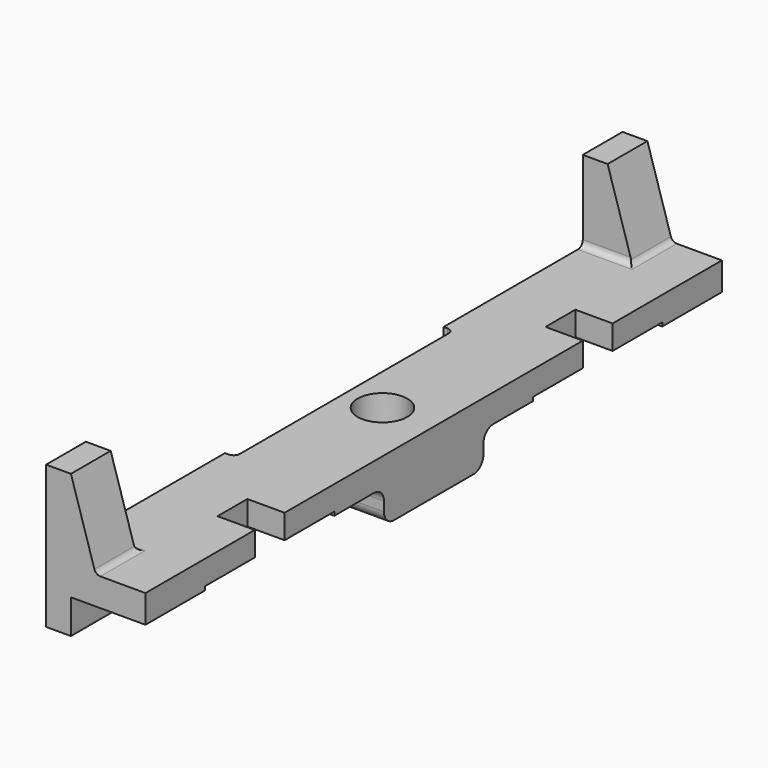
from build123d import *

# Parameters (mm, degrees)
F0_W      = 58
F0_H      = 5
F1_DEPTH  = 2
F2_W      = 13
F2_H      = 0.5
F3_DEPTH  = 0.8
F4_W      = 58
F4_H      = 2.25
F5_DEPTH  = 6
F6_W      = 6
F6_H      = 10
F7_DEPTH  = 2.75
F8_R      = 2
F9_DEPTH  = 4
F10_R     = 1
F12_DEPTH = 4
F13_W     = 22
F13_H     = 5
F14_DEPTH = 0.8
F15_R     = 0.5
F16_W     = 6.8
F16_H     = 13
F17_DEPTH = 0.3
F18_W     = 3
F18_H     = 3
F19_DEPTH = 1.95


# Not quite as in the source:
# - a pattern or mirror of a feature is missing from the dataset's text; its kind, count and spacing are read off the source's solid


with BuildPart() as f1:
    # F0 (on Right) → F1 (new body)
    with BuildSketch(Plane.YZ):
        Rectangle(F0_W, F0_H)
    extrude(amount=F1_DEPTH)

    # F2 (on face) → F3 (cut)
    with BuildSketch(Plane.YZ.offset(2)):
        with Locations((16.5, 0)):
            Rectangle(F2_W, F2_H)
        with Locations((-16.5, 0)):
            Rectangle(F2_W, F2_H)
    extrude(amount=-F3_DEPTH, mode=Mode.SUBTRACT)

    # F4 (on face) → F5 (join)
    with BuildSketch(Plane.YZ.offset(2)):
        with Locations((0, 1.375)):
            Rectangle(F4_W, F4_H)
    extrude(amount=F5_DEPTH)

    # F6 (on face) → F7 (join, through all)
    with BuildSketch(Plane(origin=(0, 0, 0.25), x_dir=(1, 0, 0), z_dir=(0, 0, -1))):
        with Locations((5, 0)):
            Rectangle(F6_W, F6_H)
    extrude(amount=F7_DEPTH)

    # F8 (on face) → F9 (cut)
    with BuildSketch(Plane.XY.offset(2.5)):
        with Locations((3.875, 0)):
            Circle(F8_R)
    extrude(amount=-F9_DEPTH, mode=Mode.SUBTRACT)

    # F10
    f10_edges = [f1.edges().sort_by_distance(p)[0] for p in [
        (5, -5, -2.5),
        (5, -5, 0.25),
        (5, 5, 0.25),
        (5, 5, -2.5),
    ]]
    fillet(f10_edges, radius=F10_R)

    # F11 (on face) → F12 (join)
    with BuildSketch(Plane(origin=(0, 29, 0), x_dir=(-1, 0, 0), z_dir=(0, 1, 0))):
        Polygon((-4, 2.5), (0, 2.5), (0, 9), (-2, 9), align=None)
    f12 = extrude(amount=-F12_DEPTH)

    # F12_copies: F12 across plane
    add(f12.mirror(Plane(origin=(0, 0, 0), x_dir=(0, 0, -1), z_dir=(0, -1, 0))))

    # F13 (on face) → F14 (cut)
    with BuildSketch(Plane(origin=(0, 0, 0), x_dir=(0, -1, 0), z_dir=(-1, 0, 0))):
        Rectangle(F13_W, F13_H)
    extrude(amount=-F14_DEPTH, mode=Mode.SUBTRACT)

    # F15
    f15_edges = [f1.edges().sort_by_distance(p)[0] for p in [
        (0.8, 11, 0),
        (0.8, -11, 0),
        (4, 27, 2.5),
        (2, 25, 2.5),
        (2, -25, 2.5),
        (4, -27, 2.5),
    ]]
    fillet(f15_edges, radius=F15_R)

    # F16 (on face) → F17 (cut)
    with BuildSketch(Plane(origin=(0, 0, 0.25), x_dir=(1, 0, 0), z_dir=(0, 0, -1))):
        with Locations((4.6, 16.5)):
            Rectangle(F16_W, F16_H)
        with Locations((4.6, -16.5)):
            Rectangle(F16_W, F16_H)
    extrude(amount=-F17_DEPTH, mode=Mode.SUBTRACT)

    # F18 (on face) → F19 (cut, through all)
    with BuildSketch(Plane(origin=(0, 0, 0.55), x_dir=(1, 0, 0), z_dir=(0, 0, -1))):
        with Locations((6.5, -16.5)):
            Rectangle(F18_W, F18_H)
        with Locations((6.5, 16.5)):
            Rectangle(F18_W, F18_H)
    extrude(amount=-F19_DEPTH, mode=Mode.SUBTRACT)


solid = f1.part
